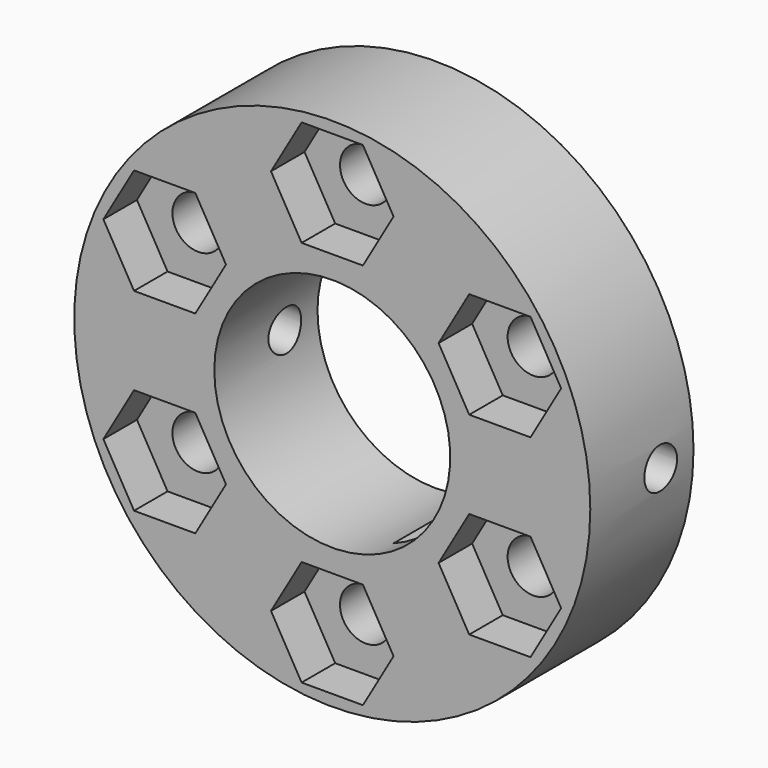
from build123d import *

# Parameters (mm, degrees)
F0_R            = 20
F1_DEPTH        = 10
F3_DEPTH        = 8.5
F4_R            = 2
F5_DEPTH        = 10.001
F5_COPIES_COUNT = 6
F7_DEPTH        = 3.25
F7_COPIES_COUNT = 6
F8_R            = 5.08
F9_DEPTH        = 10.001
F10_R           = 9.144
F11_DEPTH       = 10.001
F13_DEPTH       = 8.128
F14_R           = 1.5875
F15_DEPTH       = 25.4


# Not quite as in the source:
# - a pattern or mirror of a feature is missing from the dataset's text; its kind, count and spacing are read off the source's solid


with BuildPart() as f1:
    # F0 (on Front) → F1 (new body)
    with BuildSketch(Plane.XZ):
        Circle(F0_R)
    extrude(amount=F1_DEPTH)

    # F2 (on face) → F3 (cut)
    with BuildSketch(Plane(origin=(0, 0, 0), x_dir=(-1, 0, 0), z_dir=(0, 1, 0))):
        Polygon((3.3197640478, 5.75), (-3.3197640478, 5.75), (-6.6395280957, 0), (-3.3197640478, -5.75), (3.3197640478, -5.75), (6.6395280957, 0), align=None)
    extrude(amount=-F3_DEPTH, mode=Mode.SUBTRACT)

    # F4 (on face) → F5 (cut, through all)
    with BuildSketch(Plane.XZ.offset(10)):
        with Locations((0, 15)):
            Circle(F4_R)
    f5 = extrude(amount=-F5_DEPTH, mode=Mode.SUBTRACT)

    # F5_copies: F5 ×6 about axis
    f5_copies_axis = Axis((0, 0, 0), (0, 1, 0))
    for i in range(1, F5_COPIES_COUNT):
        add(f5.rotate(f5_copies_axis, i * 360 / F5_COPIES_COUNT), mode=Mode.SUBTRACT)

    # F6 (on face) → F7 (cut)
    with BuildSketch(Plane.XZ.offset(10)):
        Polygon((2.375, 19.113620668), (-2.375, 19.113620668), (-4.75, 15), (-2.375, 10.886379332), (2.375, 10.886379332), (4.75, 15), align=None)
    f7 = extrude(amount=-F7_DEPTH, mode=Mode.SUBTRACT)

    # F7_copies: F7 ×6 about axis
    f7_copies_axis = Axis((0, 0, 0), (0, 1, 0))
    for i in range(1, F7_COPIES_COUNT):
        add(f7.rotate(f7_copies_axis, i * 360 / F7_COPIES_COUNT), mode=Mode.SUBTRACT)

    # F8 (on face) → F9 (cut, through all)
    with BuildSketch(Plane.XZ.offset(10)):
        Circle(F8_R)
    extrude(amount=-F9_DEPTH, mode=Mode.SUBTRACT)

    # F10 (on face) → F11 (cut, through all)
    with BuildSketch(Plane(origin=(0, 0, 0), x_dir=(-1, 0, 0), z_dir=(0, 1, 0))):
        Circle(F10_R)
    extrude(amount=-F11_DEPTH, mode=Mode.SUBTRACT)

    # F12 (on face) → F13 (cut)
    with BuildSketch(Plane(origin=(0, 0, 0), x_dir=(-1, 0, 0), z_dir=(0, 1, 0))):
        Polygon((9.2023301022, 13.0179032851), (6.6726698978, 14.4784032851), (-9.2023301022, -13.0179032851), (-6.6726698978, -14.4784032851), align=None)
    extrude(amount=-F13_DEPTH, mode=Mode.SUBTRACT)

    # F14 (on Right) → F15 (cut, symmetric)
    with BuildSketch(Plane.YZ):
        with Locations((-3.175, 0)):
            Circle(F14_R)
    extrude(amount=F15_DEPTH, both=True, mode=Mode.SUBTRACT)


solid = f1.part
